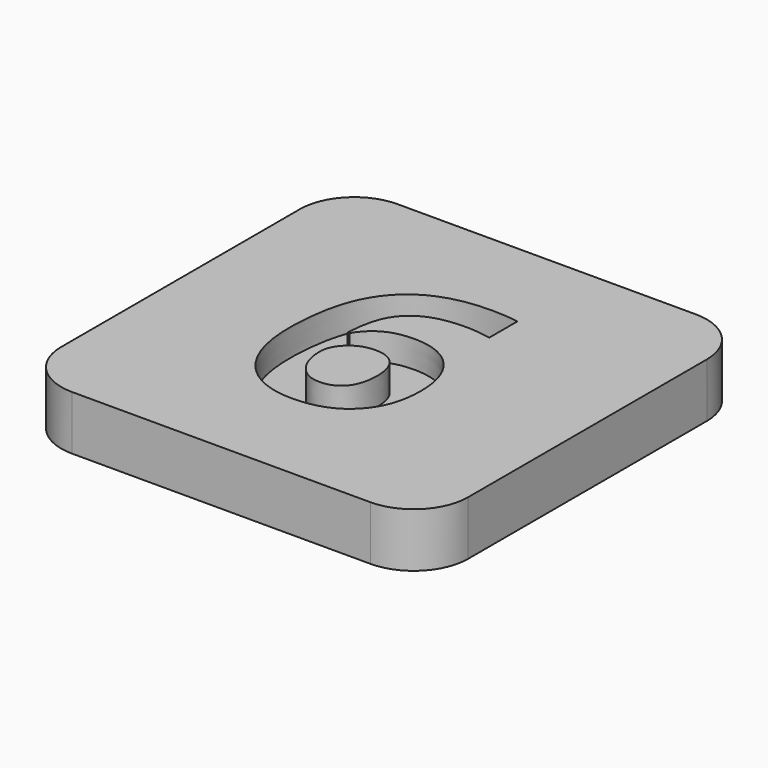
from build123d import *

# Parameters (mm, degrees)
F0_W         = 38.1
F0_H         = 38.1
F1_DEPTH     = 5.08
F2_TEXT_SIZE = 27.3386804657
F3_DEPTH     = 2.54
F4_R         = 5.08


# Not quite as in the source:
# - Text() gives the source's letters only with a copy of the font that has no kerning and outlines rounded to 1/6400 em; it was checked with that copy


with BuildPart() as f1:
    # F0 (on Top) → F1 (new body)
    with BuildSketch(Plane.XY):
        Rectangle(F0_W, F0_H)
    extrude(amount=F1_DEPTH)

    # F2 (on face) → F3 (cut)
    with BuildSketch(Plane.XY.offset(5.08)):
        with Locations((-8.89, -9.525)):
            Text('6', F2_TEXT_SIZE, font='Open Sans', font_style=FontStyle.BOLD, text_align=(TextAlign.LEFT, TextAlign.BOTTOM))
    extrude(amount=-F3_DEPTH, mode=Mode.SUBTRACT)

    # F4
    f4_edges = [f1.edges().sort_by_distance(p)[0] for p in [
        (-19.05, -19.05, 2.54),
        (19.05, -19.05, 2.54),
        (19.05, 19.05, 2.54),
        (-19.05, 19.05, 2.54),
    ]]
    fillet(f4_edges, radius=F4_R)


solid = f1.part
